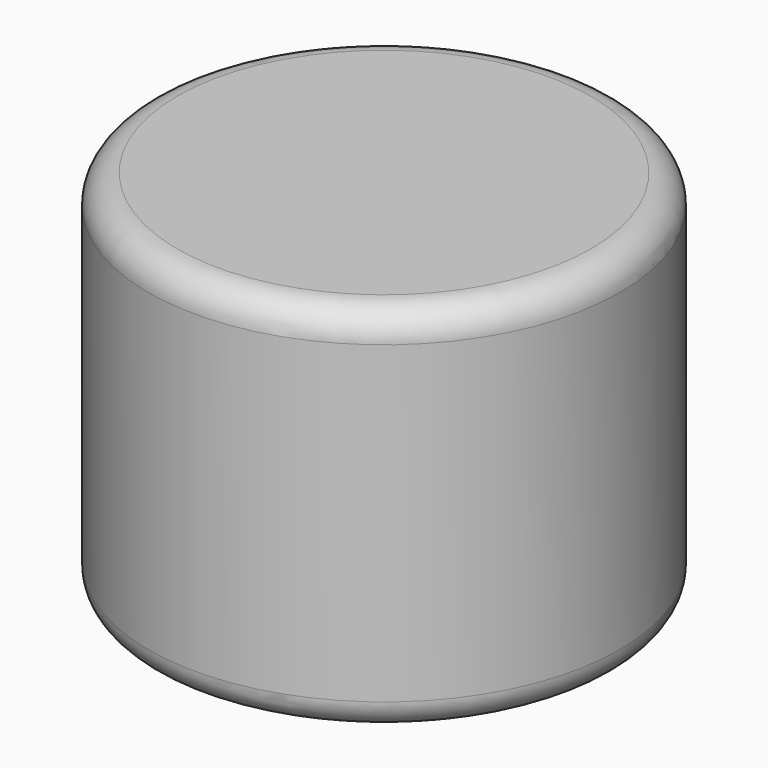
from build123d import *

# Parameters (mm, degrees)
F2_R = 0.69999
F3_R = 1


# Not quite as in the source:
# - a fillet or chamfer is up to 0.001 mm smaller than in the source, because OpenCascade refuses the exact size


with BuildPart() as f1:
    # F0 (on Front) → F1 (revolve)
    with BuildSketch(Plane.XZ):
        Polygon((0, 9), (0, 8), (4.3, 8), (4.3, 0), (5.7, 0), (5.7, 9), align=None)
    revolve(axis=Axis((0, 0, 8.5), (0, 0, -1)))

    # F2 (radius 0.7 in the source; OpenCascade refuses exactly that, so slightly less here)
    f2_edges = [f1.edges().sort_by_distance(p)[0] for p in [
        (-5.7, 0, 0),
        (-4.3, 0, 0),
        (-5.7, 0, 9),
    ]]
    fillet(f2_edges, radius=F2_R)

    # F3
    f3_edges = [f1.edges().sort_by_distance(p)[0] for p in [
        (-4.3, 0, 8),
    ]]
    fillet(f3_edges, radius=F3_R)


solid = f1.part
